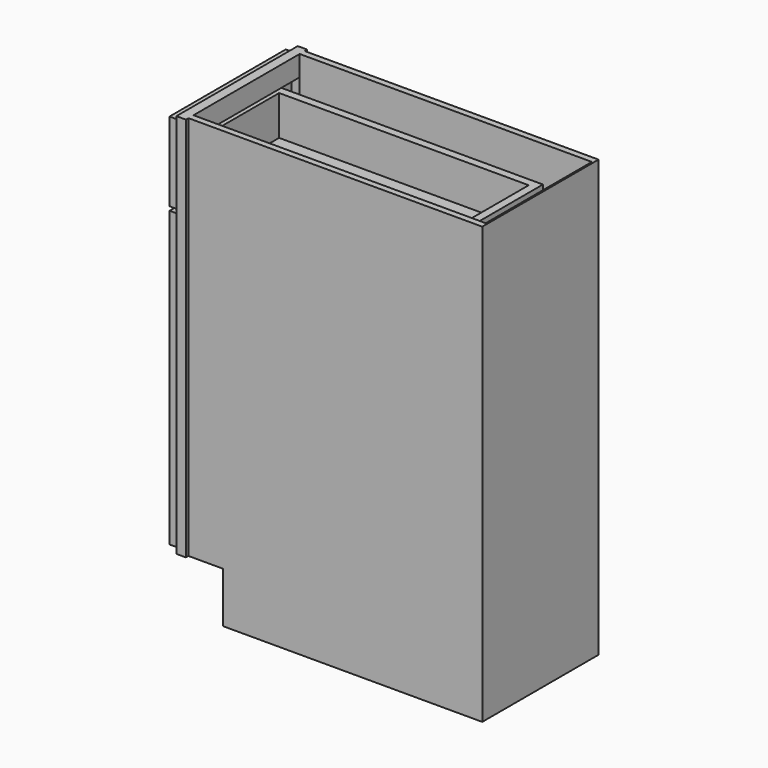
from build123d import *

# Parameters (mm, degrees)
F0_W          = 609.6
F0_H          = 876.3
F1_DEPTH      = 304.8
F2_W          = 88.9
F2_H          = 101.6
F3_DEPTH      = 304.801
F4_W          = 272.3213114754
F4_H          = 692.15
F5_DEPTH      = 19.05
F6_W          = 590.55
F6_H          = 6.35
F7_DEPTH      = 876.301
F8_W          = 587.375
F8_H          = 266.7
F9_DEPTH      = 733.425
F10_W         = 272.3213114754
F10_H         = 41.275
F11_DEPTH     = 19.05
F12_W         = 292.1
F12_H         = 590.5627
F12_W_2       = 177.8
F12_H_2       = 476.2627
F13_DEPTH     = 19.05
F14_W         = 6.35
F14_H         = 177.8
F15_DEPTH     = 476.2627
F16_SIZE      = 3.175
F17_W         = 292.1
F17_H         = 158.75
F17_W_2       = 177.8
F17_H_2       = 82.55
F18_DEPTH     = 19.05
F19_W         = 6.35
F19_H         = 177.8
F20_DEPTH     = 82.55
F21_SIZE      = 3.175
F22_W         = 504.825
F22_H         = 266.7
F23_DEPTH     = 101.6
F24_W         = 203.2
F24_H         = 95.25
F25_DEPTH     = 533.4
F26_T         = 15.875
F26_T3_DEPTH  = 37.249261314
F26_T5_DEPTH  = 37.249261314
F26_T7_DEPTH  = 37.249261314
F26_T9_DEPTH  = 37.249261314
F26_T11_DEPTH = 36.5125
F26_T13_DEPTH = 209.55
F26_T15_DEPTH = 114.3
F26_T17_DEPTH = 127
F26_T19_DEPTH = 234.95
F26_T21_DEPTH = 111.125
F26_T23_DEPTH = 36.5125


# Not quite as in the source:
# - a shell that OpenCascade refuses in one call is made with other operations: the cavity is built on its own and cut out


with BuildPart() as f1:
    # F0 (on Front) → F1 (new body)
    with BuildSketch(Plane.XZ):
        Rectangle(F0_W, F0_H)
    extrude(amount=-F1_DEPTH)

    # F2 (on face) → F3 (cut, through all)
    with BuildSketch(Plane.XZ):
        with Locations((-260.35, -387.35)):
            Rectangle(F2_W, F2_H)
    extrude(amount=-F3_DEPTH, mode=Mode.SUBTRACT)

    # F4 (on face) → F5 (cut)
    with BuildSketch(Plane(origin=(-304.8, 0, 0), x_dir=(0, -1, 0), z_dir=(-1, 0, 0))):
        with Locations((-152.4, 50.8)):
            Rectangle(F4_W, F4_H)
    extrude(amount=-F5_DEPTH, mode=Mode.SUBTRACT)

    # F6 (on face) → F7 (cut, through all)
    with BuildSketch(Plane.XY.offset(438.15)):
        with Locations((9.525, 301.625)):
            Rectangle(F6_W, F6_H)
        with Locations((9.525, 3.175)):
            Rectangle(F6_W, F6_H)
    extrude(amount=-F7_DEPTH, mode=Mode.SUBTRACT)

    # F8 (on face) → F9 (cut, through all)
    with BuildSketch(Plane.XY.offset(438.15)):
        with Locations((7.9375, 152.4)):
            Rectangle(F8_W, F8_H)
    extrude(amount=-F9_DEPTH, mode=Mode.SUBTRACT)

    # F10 (on face) → F11 (join, through all)
    with BuildSketch(Plane(origin=(-304.8, 0, 0), x_dir=(0, -1, 0), z_dir=(-1, 0, 0))):
        with Locations((-152.4, 265.1125)):
            Rectangle(F10_W, F10_H)
    extrude(amount=-F11_DEPTH)

    # F22 (on face) → F23 (cut)
    with BuildSketch(Plane(origin=(0, 0, -438.15), x_dir=(1, 0, 0), z_dir=(0, 0, -1))):
        with Locations((49.2125, -152.4)):
            Rectangle(F22_W, F22_H)
    extrude(amount=-F23_DEPTH, mode=Mode.SUBTRACT)


with BuildPart() as f13:
    # F12 (on face) → F13 (new body)
    with BuildSketch(Plane(origin=(-304.8, 0, 0), x_dir=(0, -1, 0), z_dir=(-1, 0, 0))):
        with Locations((-152.4, -33.33115)):
            Rectangle(F12_W, F12_H)
        with Locations((-152.4, -33.33115)):
            Rectangle(F12_W_2, F12_H_2, mode=Mode.SUBTRACT)
    extrude(amount=F13_DEPTH)

    # F14 (on face) → F15 (join, through all)
    with BuildSketch(Plane.XY.offset(-271.4625)):
        with Locations((-312.7375, 152.4)):
            Rectangle(F14_W, F14_H)
    extrude(amount=F15_DEPTH)

    # F16
    f16_edges = [f13.edges().sort_by_distance(p)[0] for p in [
        (-323.85, 241.3, -33.33115),
        (-323.85, 152.4, -271.4625),
        (-323.85, 63.5, -33.33115),
        (-323.85, 152.4, 204.8002),
    ]]
    chamfer(f16_edges, length=F16_SIZE)


with BuildPart() as f18:
    # F17 (on face) → F18 (new body)
    with BuildSketch(Plane(origin=(-304.8, 0, 0), x_dir=(0, -1, 0), z_dir=(-1, 0, 0))):
        with Locations((-152.4, 349.25)):
            Rectangle(F17_W, F17_H)
        with Locations((-152.4, 349.25)):
            Rectangle(F17_W_2, F17_H_2, mode=Mode.SUBTRACT)
    extrude(amount=F18_DEPTH)

    # F19 (on face) → F20 (join, through all)
    with BuildSketch(Plane.XY.offset(307.975)):
        with Locations((-312.7375, 152.4)):
            Rectangle(F19_W, F19_H)
    extrude(amount=F20_DEPTH)

    # F21
    f21_edges = [f18.edges().sort_by_distance(p)[0] for p in [
        (-323.85, 152.4, 307.975),
        (-323.85, 241.3, 349.25),
        (-323.85, 152.4, 390.525),
        (-323.85, 63.5, 349.25),
    ]]
    chamfer(f21_edges, length=F21_SIZE)

    # F24 (on face) → F25 (join)
    with BuildSketch(Plane.YZ.offset(-304.8)):
        with Locations((152.4, 339.725)):
            Rectangle(F24_W, F24_H)
    extrude(amount=F25_DEPTH)

    # F26: shell of thickness 15.875, made by hand


with BuildPart() as f26_core1:
    # F26_t2: copy of F18
    add(f18.part)

    # the walls: a layer under each face that stays
    f26_faces = [f26_core1.faces().sort_by_distance(p)[0] for p in [
        (-323.85, 249.7666666667, 296.3333333333),
        (-322.2625, 152.4, 306.3875),
        (-322.2625, 61.9125, 349.25),
        (-322.2625, 242.8875, 349.25),
        (-322.2625, 152.4, 392.1125),
        (-314.325, 152.4, 428.625),
        (-314.325, 298.45, 349.25),
        (-314.325, 152.4, 269.875),
        (-314.325, 6.35, 349.25),
        (-318.29375, 152.4, 307.975),
        (-318.29375, 63.5, 349.25),
        (-318.29375, 241.3, 349.25),
        (-318.29375, 152.4, 390.525),
        (-304.8, 249.7666666667, 402.1666666667),
        (-315.9125, 152.4, 349.25),
        (-38.1, 254, 339.725),
        (-38.1, 152.4, 292.1),
        (-38.1, 50.8, 339.725),
        (-307.18125, 63.5, 349.25),
        (-307.18125, 152.4, 390.525),
        (-307.18125, 241.3, 349.25),
        (-304.8, 152.4, 347.6625),
        (228.6, 152.4, 339.725),
        (-307.18125, 152.4, 307.975),
        (-309.5625, 152.4, 349.25),
    ]]
    thicken(f26_faces, amount=-F26_T, mode=Mode.SUBTRACT)

    # F26_s4 → F26_t3 (cut)
    with BuildSketch(Plane(origin=(4.5928978099, 4.5928978099, 4.5928978099), x_dir=(-0.7071067812, 0.7071067812, 0), z_dir=(0.5773502692, 0.5773502692, 0.5773502692))):
        Polygon((271.8908726623, 356.5892701441), (263.7152476623, 342.7036353262), (255.7777476623, 347.2863530879), (255.7777476623, 356.4517886113), align=None)
    extrude(amount=F26_T3_DEPTH, mode=Mode.SUBTRACT)

    # F26_s6 → F26_t5 (cut)
    with BuildSketch(Plane(origin=(-97.0071021901, 97.0071021901, -97.0071021901), x_dir=(0.7071067812, 0.7071067812, 0), z_dir=(0.5773502692, -0.5773502692, 0.5773502692))):
        Polygon((-56.3647257567, 481.0233490775), (-48.1891007567, 467.1377142596), (-40.2516007567, 471.7204320213), (-40.2516007567, 480.8858675446), align=None)
    extrude(amount=F26_T5_DEPTH, mode=Mode.SUBTRACT)

    # F26_s8 → F26_t7 (cut)
    with BuildSketch(Plane(origin=(-228.2404355234, -228.2404355234, 228.2404355234), x_dir=(-0.7071067812, 0.7071067812, 0), z_dir=(0.5773502692, 0.5773502692, -0.5773502692))):
        Polygon((271.8908726623, 213.7335916339), (255.7777476623, 213.8710731668), (255.7777476623, 223.0365086901), (263.7152476623, 227.6192264518), align=None)
    extrude(amount=F26_T7_DEPTH, mode=Mode.SUBTRACT)

    # F26_s10 → F26_t9 (cut)
    with BuildSketch(Plane(origin=(-329.8404355234, 329.8404355234, 329.8404355234), x_dir=(0.7071067812, 0.7071067812, 0), z_dir=(0.5773502692, -0.5773502692, -0.5773502692))):
        Polygon((-56.3647257567, 89.2995127005), (-40.2516007567, 89.4369942334), (-40.2516007567, 98.6024297568), (-48.1891007567, 103.1851475184), align=None)
    extrude(amount=F26_T9_DEPTH, mode=Mode.SUBTRACT)

    # F26_s12 → F26_t11 (cut)
    with BuildSketch(Plane.YZ.offset(-336.55)):
        Polygon((241.14125, 308.13375), (241.3, 292.1), (257.175, 292.1), (257.175, 307.975), align=None)
        Polygon((63.65875, 308.13375), (63.5, 292.1), (47.625, 292.1), (47.625, 307.975), align=None)
        Polygon((63.65875, 390.36625), (47.625, 390.525), (47.625, 406.4), (63.5, 406.4), align=None)
        Polygon((241.14125, 390.36625), (257.175, 390.525), (257.175, 406.4), (241.3, 406.4), align=None)
    extrude(amount=F26_T11_DEPTH, mode=Mode.SUBTRACT)

    # F26_s14 → F26_t13 (cut)
    with BuildSketch(Plane.XZ.offset(-257.175)):
        Polygon((-316.07125, 308.13375), (-315.9125, 292.1), (-300.0375, 292.1), (-300.0375, 307.975), align=None)
        Polygon((-316.07125, 390.36625), (-315.9125, 406.4), (-300.0375, 406.4), (-300.0375, 390.525), align=None)
        Polygon((-309.40375, 390.36625), (-309.5625, 406.4), (-325.4375, 406.4), (-325.4375, 390.525), align=None)
        Polygon((-304.95875, 308.13375), (-288.925, 307.975), (-288.925, 292.1), (-304.8, 292.1), align=None)
        Polygon((-309.40375, 308.13375), (-309.5625, 292.1), (-325.4375, 292.1), (-325.4375, 307.975), align=None)
    extrude(amount=F26_T13_DEPTH, mode=Mode.SUBTRACT)

    # F26_s16 → F26_t15 (cut)
    with BuildSketch(Plane.XY.offset(292.1)):
        Polygon((-316.07125, 63.65875), (-315.9125, 47.625), (-300.0375, 47.625), (-300.0375, 63.5), align=None)
        Polygon((-316.07125, 241.14125), (-315.9125, 257.175), (-300.0375, 257.175), (-300.0375, 241.3), align=None)
        Polygon((-309.40375, 63.65875), (-309.5625, 47.625), (-325.4375, 47.625), (-325.4375, 63.5), align=None)
        Polygon((-309.40375, 241.14125), (-309.5625, 257.175), (-325.4375, 257.175), (-325.4375, 241.3), align=None)
    extrude(amount=F26_T15_DEPTH, mode=Mode.SUBTRACT)

    # F26_s18 → F26_t17 (cut)
    with BuildSketch(Plane.XY.offset(276.225)):
        Polygon((-304.64125, 254.15875), (-320.675, 254), (-320.675, 238.125), (-304.8, 238.125), align=None)
        Polygon((-304.64125, 50.64125), (-320.675, 50.8), (-320.675, 66.675), (-304.8, 66.675), align=None)
    extrude(amount=F26_T17_DEPTH, mode=Mode.SUBTRACT)

    # F26_s20 → F26_t19 (cut)
    with BuildSketch(Plane.XZ.offset(-269.875)):
        Polygon((-304.64125, 291.94125), (-320.675, 292.1), (-320.675, 307.975), (-304.8, 307.975), align=None)
    extrude(amount=F26_T19_DEPTH, mode=Mode.SUBTRACT)

    # F26_s22 → F26_t21 (cut)
    with BuildSketch(Plane.XY.offset(292.1)):
        Polygon((-304.95875, 63.65875), (-304.8, 47.625), (-288.925, 47.625), (-288.925, 63.5), align=None)
        Polygon((-304.95875, 241.14125), (-304.8, 257.175), (-288.925, 257.175), (-288.925, 241.3), align=None)
    extrude(amount=F26_T21_DEPTH, mode=Mode.SUBTRACT)

    # F26_s24 → F26_t23 (cut)
    with BuildSketch(Plane.YZ.offset(-325.4375)):
        Polygon((63.65875, 308.13375), (47.625, 307.975), (47.625, 292.1), (63.5, 292.1), align=None)
        Polygon((63.65875, 390.36625), (47.625, 390.525), (47.625, 406.4), (63.5, 406.4), align=None)
        Polygon((241.14125, 390.36625), (241.3, 406.4), (257.175, 406.4), (257.175, 390.525), align=None)
        Polygon((241.14125, 308.13375), (257.175, 307.975), (257.175, 292.1), (241.3, 292.1), align=None)
    extrude(amount=F26_T23_DEPTH, mode=Mode.SUBTRACT)


with BuildPart() as f18_1:
    add(f18.part)

    # what is left inside the walls is the cavity
    f26_cavity = [f26_core1.part.solids().sort_by_distance(p)[0] for p in [
        (45.508333, 152.4, 308.13375),
    ]]
    add(f26_cavity, mode=Mode.SUBTRACT)


solid = Compound([f1.part, f13.part, f18_1.part])
